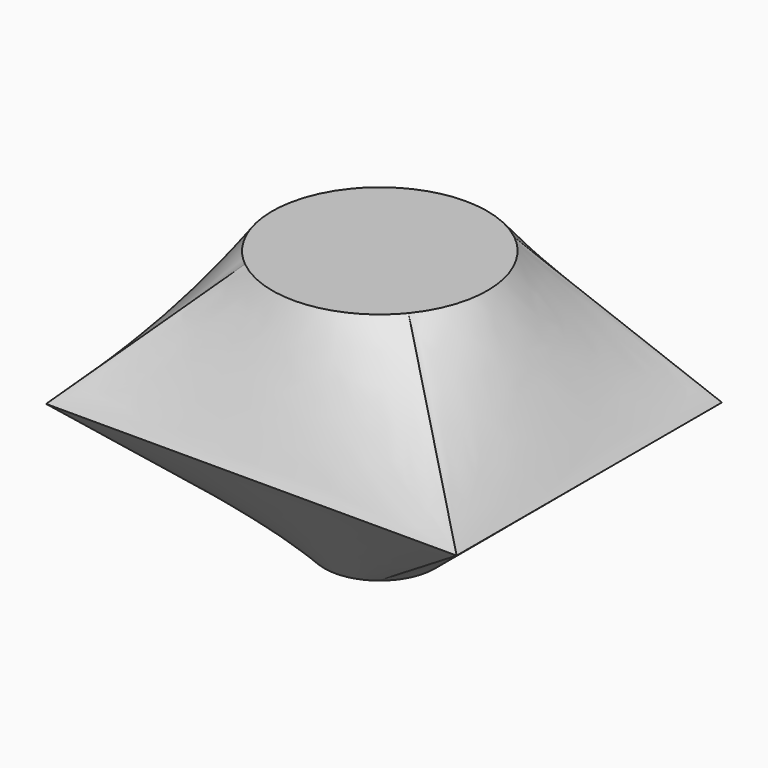
from build123d import *

# Parameters (mm, degrees)
F3_W      = 79.7774158418
F3_H      = 64.4266568124
F5_FACE_W = 79.7774158418
F5_FACE_H = 64.4266568124


# Not quite as in the source:
# - the arcs of a loft's sections are written as splines that run evenly, so that the points pair up as in the source's solid


with BuildPart() as f5:
    # F3 (on offset) → F5 section 0
    with BuildSketch(Plane.XY.offset(25.4)):
        with Locations((1.2792292982, -0.5814675242)):
            Rectangle(F3_W, F3_H)
    # F2 (on offset) → F5 section 1
    with BuildSketch(Plane.XY.offset(50.8)):
        with BuildLine():
            add(Edge.make_bspline(
                [(-16.1724337652, 13.2497043015), (-17.0396248839, 12.1912209867), (-17.8025456302, 11.0473550868), (-19.0906024978, 8.6327041883), (-19.6157067692, 7.3619788968), (-20.4079389638, 4.7424374092), (-20.6750472976, 3.3936859865), (-20.9410097804, 0.6699214201), (-20.939857353, -0.7050243732), (-20.6693293349, -3.4283392736), (-20.3999604336, -4.7766410415), (-19.6033381546, -7.3948508116), (-19.0761044751, -8.6646940734), (-17.7840016828, -11.0771823799), (-17.0191645197, -12.2197677712), (-15.2812359996, -14.3338240416), (-14.3081876162, -15.3052426465), (-13.2497043015, -16.1724337652)],
                knots=[0, 0, 0, 0, 0.125, 0.125, 0.25, 0.25, 0.375, 0.375, 0.5, 0.5, 0.625, 0.625, 0.75, 0.75, 0.875, 0.875, 1, 1, 1, 1], degree=3))
            add(Edge.make_bspline(
                [(-13.2497043015, -16.1724337652), (-12.1912209867, -17.0396248839), (-11.0473550868, -17.8025456302), (-8.6327041883, -19.0906024978), (-7.3619788968, -19.6157067692), (-4.7424374092, -20.4079389638), (-3.3936859865, -20.6750472976), (-0.6699214201, -20.9410097804), (0.7050243732, -20.939857353), (3.4283392736, -20.6693293349), (4.7766410415, -20.3999604336), (7.3948508116, -19.6033381546), (8.6646940734, -19.0761044751), (11.0771823799, -17.7840016828), (12.2197677712, -17.0191645197), (14.3338240416, -15.2812359996), (15.3052426465, -14.3081876162), (16.1724337652, -13.2497043015)],
                knots=[0, 0, 0, 0, 0.125, 0.125, 0.25, 0.25, 0.375, 0.375, 0.5, 0.5, 0.625, 0.625, 0.75, 0.75, 0.875, 0.875, 1, 1, 1, 1], degree=3))
            add(Edge.make_bspline(
                [(16.1724337652, -13.2497043015), (17.0396248839, -12.1912209867), (17.8025456302, -11.0473550868), (19.0906024978, -8.6327041883), (19.6157067692, -7.3619788968), (20.4079389638, -4.7424374092), (20.6750472976, -3.3936859865), (20.9410097804, -0.6699214201), (20.939857353, 0.7050243732), (20.6693293349, 3.4283392736), (20.3999604336, 4.7766410415), (19.6033381546, 7.3948508116), (19.0761044751, 8.6646940734), (17.7840016828, 11.0771823799), (17.0191645197, 12.2197677712), (15.2812359996, 14.3338240416), (14.3081876162, 15.3052426465), (13.2497043015, 16.1724337652)],
                knots=[0, 0, 0, 0, 0.125, 0.125, 0.25, 0.25, 0.375, 0.375, 0.5, 0.5, 0.625, 0.625, 0.75, 0.75, 0.875, 0.875, 1, 1, 1, 1], degree=3))
            add(Edge.make_bspline(
                [(13.2497043015, 16.1724337652), (12.1912209867, 17.0396248839), (11.0473550868, 17.8025456302), (8.6327041883, 19.0906024978), (7.3619788968, 19.6157067692), (4.7424374092, 20.4079389638), (3.3936859865, 20.6750472976), (0.6699214201, 20.9410097804), (-0.7050243732, 20.939857353), (-3.4283392736, 20.6693293349), (-4.7766410415, 20.3999604336), (-7.3948508116, 19.6033381546), (-8.6646940734, 19.0761044751), (-11.0771823799, 17.7840016828), (-12.2197677712, 17.0191645197), (-14.3338240416, 15.2812359996), (-15.3052426465, 14.3081876162), (-16.1724337652, 13.2497043015)],
                knots=[0, 0, 0, 0, 0.125, 0.125, 0.25, 0.25, 0.375, 0.375, 0.5, 0.5, 0.625, 0.625, 0.75, 0.75, 0.875, 0.875, 1, 1, 1, 1], degree=3))
        make_face()
    loft(ruled=True)

    # F5_face (on face) → F6 section 0
    with BuildSketch(Plane(origin=(1.2792292982, -0.5814675242, 25.4), x_dir=(1, 0, 0), z_dir=(0, 0, -1))):
        Rectangle(F5_FACE_W, F5_FACE_H)
    # F4 (on Top) → F6 section 1
    with BuildSketch(Plane.XY):
        with BuildLine():
            add(Edge.make_bspline(
                [(8.5557200784, 6.5738865133), (7.6952003461, 7.6938276526), (6.6123366987, 8.6422274732), (4.1651377242, 10.0529955761), (2.8017652653, 10.5148087816), (0.0009706408, 10.8816860538), (-1.4353495317, 10.78660577), (-4.1633442138, 10.0537384724), (-5.4539453739, 9.4162398107), (-6.5738865133, 8.5557200784)],
                knots=[0, 0, 0, 0, 0.25, 0.25, 0.5, 0.5, 0.75, 0.75, 1, 1, 1, 1], degree=3))
            add(Edge.make_bspline(
                [(-6.5738865133, 8.5557200784), (-7.6938276526, 7.6952003461), (-8.6422274732, 6.6123366987), (-10.0529955761, 4.1651377242), (-10.5148087816, 2.8017652653), (-10.8816860538, 0.0009706408), (-10.78660577, -1.4353495317), (-10.0537384724, -4.1633442138), (-9.4162398107, -5.4539453739), (-8.5557200784, -6.5738865133)],
                knots=[0, 0, 0, 0, 0.25, 0.25, 0.5, 0.5, 0.75, 0.75, 1, 1, 1, 1], degree=3))
            add(Edge.make_bspline(
                [(-8.5557200784, -6.5738865133), (-7.6952003461, -7.6938276526), (-6.6123366987, -8.6422274732), (-4.1651377242, -10.0529955761), (-2.8017652653, -10.5148087816), (-0.0009706408, -10.8816860538), (1.4353495317, -10.78660577), (4.1633442138, -10.0537384724), (5.4539453739, -9.4162398107), (6.5738865133, -8.5557200784)],
                knots=[0, 0, 0, 0, 0.25, 0.25, 0.5, 0.5, 0.75, 0.75, 1, 1, 1, 1], degree=3))
            add(Edge.make_bspline(
                [(6.5738865133, -8.5557200784), (7.6938276526, -7.6952003461), (8.6422274732, -6.6123366987), (10.0529955761, -4.1651377242), (10.5148087816, -2.8017652653), (10.8816860538, -0.0009706408), (10.78660577, 1.4353495317), (10.0537384724, 4.1633442138), (9.4162398107, 5.4539453739), (8.5557200784, 6.5738865133)],
                knots=[0, 0, 0, 0, 0.25, 0.25, 0.5, 0.5, 0.75, 0.75, 1, 1, 1, 1], degree=3))
        make_face()
    loft(ruled=True)


solid = f5.part
